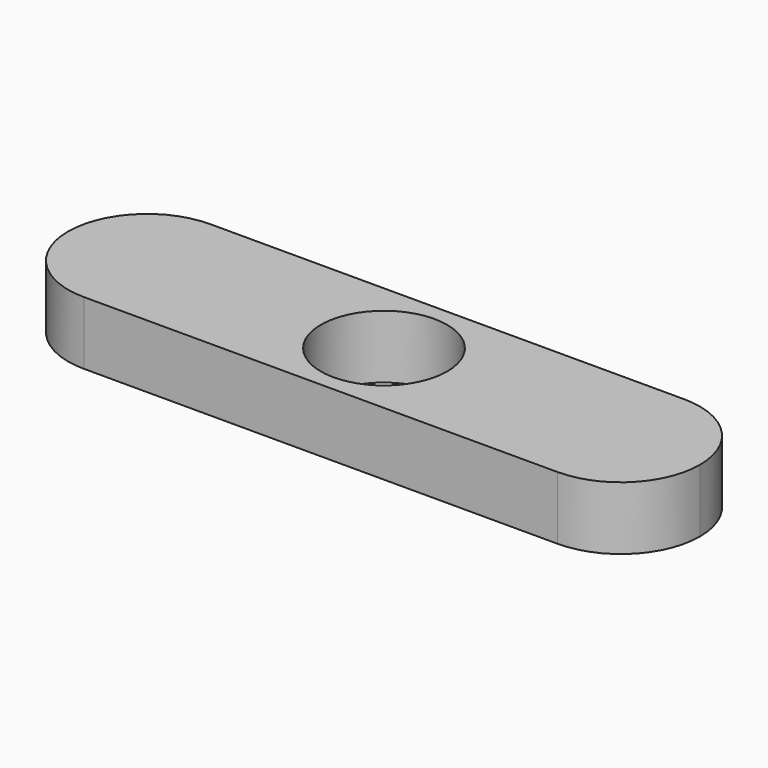
from build123d import *

# Parameters (mm, degrees)
F0_W     = 200
F0_H     = 50
F0_R     = 20
F1_DEPTH = 20
F2_R     = 24.99999


# Not quite as in the source:
# - a fillet or chamfer is up to 0.001 mm smaller than in the source, because OpenCascade refuses the exact size


with BuildPart() as f1:
    # F0 (on Top) → F1 (new body)
    with BuildSketch(Plane.XY):
        with Locations((100, 25)):
            Rectangle(F0_W, F0_H)
        with Locations((100, 25)):
            Circle(F0_R, mode=Mode.SUBTRACT)
    extrude(amount=F1_DEPTH)

    # F2 (radius 25 in the source; OpenCascade refuses exactly that, so slightly less here)
    f2_edges = [f1.edges().sort_by_distance(p)[0] for p in [
        (200, 0, 10),
        (0, 50, 10),
        (0, 0, 10),
        (200, 50, 10),
    ]]
    fillet(f2_edges, radius=F2_R)


solid = f1.part
